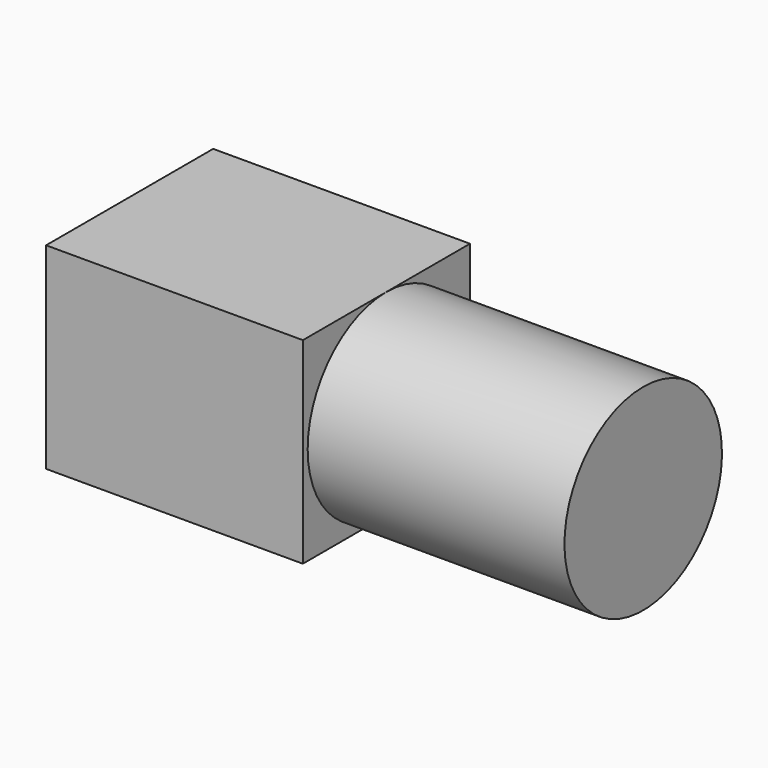
from build123d import *

# Parameters (mm, degrees)
F0_W     = 51.6446605325
F0_H     = 48.6768968403
F1_DEPTH = 63.5
F3_DEPTH = 63.5
F4_R     = 24.3384484202
F6_DEPTH = 25.399999693


# Not quite as in the source:
# - the program builds the solid bodies; features that only make, move or delete a surface that nothing else refers to are left out


with BuildPart() as f1:
    # F0 (on Right) → F1 (new body)
    with BuildSketch(Plane.YZ):
        with Locations((25.8223302662, -24.3384484202)):
            Rectangle(F0_W, F0_H)
    extrude(amount=F1_DEPTH)

    # F2 (on face) → F3 (join)
    with BuildSketch(Plane.YZ.offset(63.5)):
        with BuildLine():
            ThreePointArc((25.8223302662, -48.6768968403), (43.0322121877, -41.5483303416), (50.1607786864, -24.3384484202))
            ThreePointArc((50.1607786864, -24.3384484202), (43.0322121877, -7.1285664987), (25.8223302662, 0))
            ThreePointArc((25.8223302662, 0), (1.4838818461, -24.3384484202), (25.8223302662, -48.6768968403))
        make_face()
    extrude(amount=F3_DEPTH)

    # F4 (on face) + F5 (on face) → F6 (cut)
    with BuildSketch(Plane.YZ.offset(127)):
        with Locations((25.8223302662, -24.3384484202)):
            Circle(F4_R)
    with BuildSketch(Plane.YZ.offset(127)):
        with BuildLine():
            add(Edge.make_bspline(
                [(24.2070443928, -3.5950578749), (13.7185256549, -3.5950578749), (18.9627850239, -34.8861049861), (24.2070443928, -66.1771520972), (29.4513037618, -34.8861049861), (34.6955631307, -3.5950578749), (24.2070443928, -3.5950578749)],
                knots=[0, 0, 0, 2.0943951024, 2.0943951024, 4.1887902048, 4.1887902048, 6.2831853072, 6.2831853072, 6.2831853072], degree=2, weights=[1, 0.5, 1, 0.5, 1, 0.5, 1]))
        make_face()
    extrude(amount=F6_DEPTH, mode=Mode.SUBTRACT)


solid = f1.part
